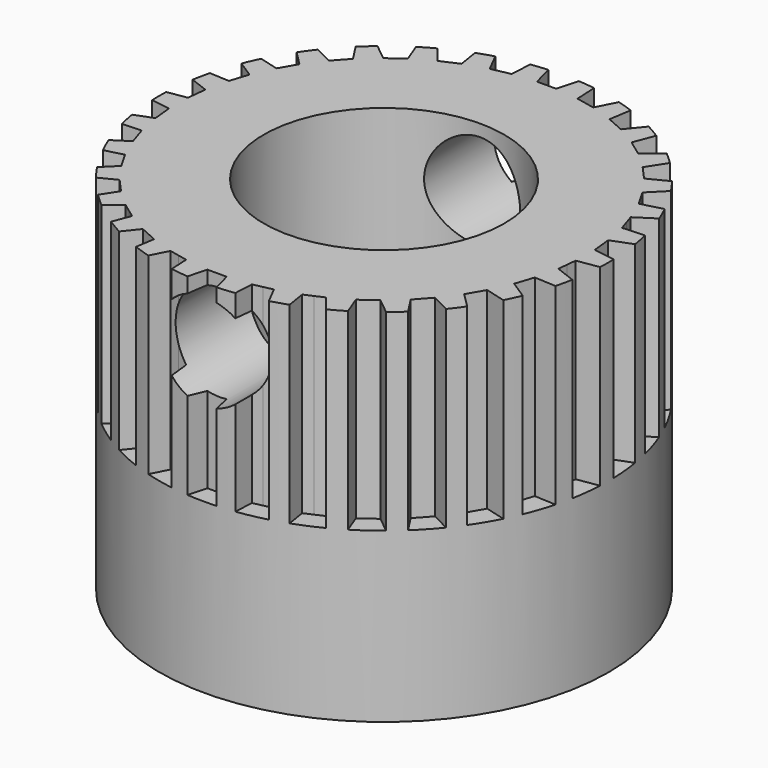
from build123d import *

# Parameters (mm, degrees)
F0_R     = 4.675
F0_R_2   = 2.5
F1_DEPTH = 7.5
F3_DEPTH = 4
F4_R     = 1
F5_DEPTH = 5


# Not quite as in the source:
# - a feature names something its author has since deleted; it is built from what else it names


with BuildPart() as f1:
    # F0 (on Top) → F1 (new body)
    with BuildSketch(Plane.XY):
        Circle(F0_R)
        Circle(F0_R_2, mode=Mode.SUBTRACT)
    extrude(amount=F1_DEPTH)

    # F2 (on face) → F3 (cut)
    with BuildSketch(Plane.XY.offset(7.5)):
        with BuildLine():
            Line((-2.705116146, -3.3310705443), (-3.0094686579, -3.5775303489))
            ThreePointArc((-3.0094686579, -3.5775303489), (-2.7721689372, -3.7643996047), (-2.5232974354, -3.9355552407))
            Line((-2.5232974354, -3.9355552407), (-2.3815093482, -3.5661846452))
            Line((-2.3815093482, -3.5661846452), (-2.5433127471, -3.4486275948))
            Line((-2.5433127471, -3.4486275948), (-2.705116146, -3.3310705443))
        make_face()
        with BuildLine():
            Line((-1.959178461, -3.8160524503), (-2.206532557, -4.12150932))
            ThreePointArc((-2.206532557, -4.12150932), (-1.9353308811, -4.2555985925), (-1.6560241348, -4.3718656275))
            Line((-1.6560241348, -4.3718656275), (-1.593760278, -3.9787471075))
            Line((-1.593760278, -3.9787471075), (-1.7764693695, -3.8973997789))
            Line((-1.7764693695, -3.8973997789), (-1.959178461, -3.8160524503))
        make_face()
        with BuildLine():
            Line((-1.1287078961, -4.1353471727), (-1.3084719445, -4.4881539825))
            ThreePointArc((-1.3084719445, -4.4881539825), (-1.0145824139, -4.5635783685), (-0.7164192765, -4.6197801268))
            Line((-0.7164192765, -4.6197801268), (-0.7374488558, -4.218511849))
            Line((-0.7374488558, -4.218511849), (-0.933078376, -4.1769295108))
            Line((-0.933078376, -4.1769295108), (-1.1287078961, -4.1353471727))
        make_face()
        with BuildLine():
            Line((-0.25, -4.275), (-0.3535915562, -4.6616089509))
            ThreePointArc((-0.3535915562, -4.6616089509), (-0.049245186, -4.6747406251), (0.2553102796, -4.6680233141))
            Line((0.2553102796, -4.6680233141), (0.15, -4.275))
            Line((0.15, -4.275), (-0.05, -4.275))
            Line((-0.05, -4.275), (-0.25, -4.275))
        make_face()
        with BuildLine():
            Line((-3.3339198947, -2.7015974913), (-3.6829835562, -2.8794543103))
            ThreePointArc((-3.6829835562, -2.8794543103), (-3.4894187684, -3.1112026065), (-3.281297254, -3.3299719715))
            Line((-3.281297254, -3.3299719715), (-3.0662676522, -2.9988554215))
            Line((-3.0662676522, -2.9988554215), (-3.2000937734, -2.8502264564))
            Line((-3.2000937734, -2.8502264564), (-3.3339198947, -2.7015974913))
        make_face()
        with BuildLine():
            Line((-3.8181079661, -1.9551442841), (-4.198151087, -2.0569765315))
            ThreePointArc((-4.198151087, -2.0569765315), (-4.0564520262, -2.3239668585), (-3.8977958923, -2.5812423718))
            Line((-3.8977958923, -2.5812423718), (-3.6181079661, -2.3015544457))
            Line((-3.6181079661, -2.3015544457), (-3.7181079661, -2.1283493649))
            Line((-3.7181079661, -2.1283493649), (-3.8181079661, -1.9551442841))
        make_face()
        with BuildLine():
            Line((-4.136519018, -1.1243345099), (-4.5325919451, -1.1450918125))
            ThreePointArc((-4.5325919451, -1.1450918125), (-4.4489051537, -1.4362687538), (-4.3465342095, -1.7214137695))
            Line((-4.3465342095, -1.7214137695), (-4.0129122202, -1.5047571164))
            Line((-4.0129122202, -1.5047571164), (-4.0747156191, -1.3145458132))
            Line((-4.0747156191, -1.3145458132), (-4.136519018, -1.1243345099))
        make_face()
        with BuildLine():
            Line((-4.2752369596, -0.2454785424), (-4.6714275586, -0.1827281161))
            ThreePointArc((-4.6714275586, -0.1827281161), (-4.6496722184, -0.4859766059), (-4.6082522435, -0.7871697783))
            Line((-4.6082522435, -0.7871697783), (-4.2334255742, -0.6432873006))
            Line((-4.2334255742, -0.6432873006), (-4.2543312669, -0.4443829215))
            Line((-4.2543312669, -0.4443829215), (-4.2752369596, -0.2454785424))
        make_face()
        with BuildLine():
            Line((-4.2281991511, 0.6430133953), (-4.6079742635, 0.7887954024))
            ThreePointArc((-4.6079742635, 0.7887954024), (-4.6496441518, 0.4862450633), (-4.6714707885, 0.1816195798))
            Line((-4.6714707885, 0.1816195798), (-4.2700105364, 0.2452046372))
            Line((-4.2700105364, 0.2452046372), (-4.2491048437, 0.4441090163))
            Line((-4.2491048437, 0.4441090163), (-4.2281991511, 0.6430133953))
        make_face()
        with BuildLine():
            Line((-3.9974613705, 1.5023099423), (-4.3441403746, 1.7274459199))
            ThreePointArc((-4.3441403746, 1.7274459199), (-4.4481636875, 1.4385634532), (-4.5329999094, 1.1434757635))
            Line((-4.5329999094, 1.1434757635), (-4.1210681683, 1.1218873357))
            Line((-4.1210681683, 1.1218873357), (-4.0592647694, 1.312098639))
            Line((-4.0592647694, 1.312098639), (-3.9974613705, 1.5023099423))
        make_face()
        with BuildLine():
            Line((-3.5931079661, 2.2948557159), (-3.8904912347, 2.5922389845))
            ThreePointArc((-3.8904912347, 2.5922389845), (-4.0531666787, 2.3296920128), (-4.198151087, 2.0569765315))
            Line((-4.198151087, 2.0569765315), (-3.7931079661, 1.9484455543))
            Line((-3.7931079661, 1.9484455543), (-3.6931079661, 2.1216506351))
            Line((-3.6931079661, 2.1216506351), (-3.5931079661, 2.2948557159))
        make_face()
        with BuildLine():
            Line((-3.0328111218, 2.9860126628), (-3.265954152, 3.3450214464))
            ThreePointArc((-3.265954152, 3.3450214464), (-3.480984636, 3.1206363075), (-3.680631567, 2.8824601069))
            Line((-3.680631567, 2.8824601069), (-3.3004633644, 2.6887547326))
            Line((-3.3004633644, 2.6887547326), (-3.1666372431, 2.8373836977))
            Line((-3.1666372431, 2.8373836977), (-3.0328111218, 2.9860126628))
        make_face()
        with BuildLine():
            Line((-2.3410584985, 3.5455739079), (-2.4971473914, 3.9521993758))
            ThreePointArc((-2.4971473914, 3.9521993758), (-2.7557916794, 3.7764053304), (-3.002104242, 3.5837124774))
            Line((-3.002104242, 3.5837124774), (-2.6646652963, 3.3104598069))
            Line((-2.6646652963, 3.3104598069), (-2.5028618974, 3.4280168574))
            Line((-2.5028618974, 3.4280168574), (-2.3410584985, 3.5455739079))
        make_face()
        with BuildLine():
            Line((-1.5480830051, 3.9490839397), (-1.6173352692, 4.3863255268))
            ThreePointArc((-1.6173352692, 4.3863255268), (-1.9086924345, 4.2676127039), (-2.1914053409, 4.1295723304))
            Line((-2.1914053409, 4.1295723304), (-1.9135011882, 3.7863892824))
            Line((-1.9135011882, 3.7863892824), (-1.7307920966, 3.8677366111))
            Line((-1.7307920966, 3.8677366111), (-1.5480830051, 3.9490839397))
        make_face()
        with BuildLine():
            Line((-0.6885414758, 4.1789074336), (-0.6650340091, 4.6274566197))
            ThreePointArc((-0.6650340091, 4.6274566197), (-0.9764656149, 4.5718858147), (-1.2834259466, 4.4953801663))
            Line((-1.2834259466, 4.4953801663), (-1.0798005161, 4.0957427572))
            Line((-1.0798005161, 4.0957427572), (-0.884170996, 4.1373250954))
            Line((-0.884170996, 4.1373250954), (-0.6885414758, 4.1789074336))
        make_face()
        with BuildLine():
            Line((0, 4.225), (0, 4.675))
            ThreePointArc((0, 4.675), (-0.1589326757, 4.672297658), (-0.3176816122, 4.664193756))
            Line((-0.3176816122, 4.664193756), (-0.2, 4.225))
            Line((-0.2, 4.225), (0, 4.225))
        make_face()
        with BuildLine():
            ThreePointArc((0.3176816122, 4.664193756), (0.1589326757, 4.672297658), (0, 4.675))
            Line((0, 4.675), (0, 4.225))
            Line((0, 4.225), (0.2, 4.225))
            Line((0.2, 4.225), (0.3176816122, 4.664193756))
        make_face()
        with BuildLine():
            ThreePointArc((1.2870955087, 4.4943308903), (0.9775168208, 4.5716611713), (0.6633841691, 4.6276934259))
            Line((0.6633841691, 4.6276934259), (0.6874488558, 4.168511849))
            Line((0.6874488558, 4.168511849), (0.883078376, 4.1269295108))
            Line((0.883078376, 4.1269295108), (1.0787078961, 4.0853471727))
            Line((1.0787078961, 4.0853471727), (1.2870955087, 4.4943308903))
        make_face()
        with BuildLine():
            ThreePointArc((2.1998941634, 4.1250564445), (1.9125739797, 4.2658745612), (1.6162943473, 4.3867091974))
            Line((1.6162943473, 4.3867091974), (1.543760278, 3.9287471075))
            Line((1.543760278, 3.9287471075), (1.7264693695, 3.8473997789))
            Line((1.7264693695, 3.8473997789), (1.909178461, 3.7660524503))
            Line((1.909178461, 3.7660524503), (2.1998941634, 4.1250564445))
        make_face()
        with BuildLine():
            ThreePointArc((3.015224498, 3.572680538), (2.763375727, 3.7708592643), (2.4985414705, 3.9513182003))
            Line((2.4985414705, 3.9513182003), (2.3315093482, 3.5161846452))
            Line((2.3315093482, 3.5161846452), (2.4933127471, 3.3986275948))
            Line((2.4933127471, 3.3986275948), (2.655116146, 3.2810705443))
            Line((2.655116146, 3.2810705443), (3.015224498, 3.572680538))
        make_face()
        with BuildLine():
            ThreePointArc((3.6966467607, 2.8618923332), (3.4918298057, 3.108496358), (3.2705945256, 3.3404844632))
            Line((3.2705945256, 3.3404844632), (3.0162676522, 2.9488554215))
            Line((3.0162676522, 2.9488554215), (3.1500937734, 2.8002264564))
            Line((3.1500937734, 2.8002264564), (3.2839198947, 2.6515974913))
            Line((3.2839198947, 2.6515974913), (3.6966467607, 2.8618923332))
        make_face()
        with BuildLine():
            ThreePointArc((4.2138675521, 2.0245852052), (4.0653705562, 2.308329968), (3.8977958923, 2.5812423718))
            Line((3.8977958923, 2.5812423718), (3.5681079661, 2.2515544457))
            Line((3.5681079661, 2.2515544457), (3.6681079661, 2.0783493649))
            Line((3.6681079661, 2.0783493649), (3.7681079661, 1.9051442841))
            Line((3.7681079661, 1.9051442841), (4.2138675521, 2.0245852052))
        make_face()
        with BuildLine():
            ThreePointArc((4.5441525528, 1.0983180672), (4.4585092177, 1.4061723064), (4.3520358228, 1.7074569386))
            Line((4.3520358228, 1.7074569386), (3.9629122202, 1.4547571164))
            Line((3.9629122202, 1.4547571164), (4.0247156191, 1.2645458132))
            Line((4.0247156191, 1.2645458132), (4.086519018, 1.0743345099))
            Line((4.086519018, 1.0743345099), (4.5441525528, 1.0983180672))
        make_face()
        with BuildLine():
            ThreePointArc((4.673341773, 0.1245057123), (4.6540213184, 0.4423918711), (4.6131030555, 0.7582250323))
            Line((4.6131030555, 0.7582250323), (4.1834255742, 0.5932873006))
            Line((4.1834255742, 0.5932873006), (4.2043312669, 0.3943829215))
            Line((4.2043312669, 0.3943829215), (4.2252369596, 0.1954785424))
            Line((4.2252369596, 0.1954785424), (4.673341773, 0.1245057123))
        make_face()
        with BuildLine():
            ThreePointArc((4.5964194804, -0.8535531385), (4.6437064147, -0.5400145687), (4.6696308942, -0.2239917685))
            Line((4.6696308942, -0.2239917685), (4.2200105364, -0.2952046372))
            Line((4.2200105364, -0.2952046372), (4.1991048437, -0.4941090163))
            Line((4.1991048437, -0.4941090163), (4.1781991511, -0.6930133953))
            Line((4.1781991511, -0.6930133953), (4.5964194804, -0.8535531385))
        make_face()
        with BuildLine():
            ThreePointArc((4.3176228817, -1.7926956383), (4.4286859235, -1.4974531683), (4.5195862819, -1.195393174))
            Line((4.5195862819, -1.195393174), (4.0710681683, -1.1718873357))
            Line((4.0710681683, -1.1718873357), (4.0092647694, -1.362098639))
            Line((4.0092647694, -1.362098639), (3.9474613705, -1.5523099423))
            Line((3.9474613705, -1.5523099423), (4.3176228817, -1.7926956383))
        make_face()
        with BuildLine():
            ThreePointArc((0.6173080827, -4.6340647094), (0.9192758993, -4.5837273938), (1.2173017982, -4.5137347432))
            Line((1.2173017982, -4.5137347432), (1.0298005161, -4.1457427572))
            Line((1.0298005161, -4.1457427572), (0.834170996, -4.1873250954))
            Line((0.834170996, -4.1873250954), (0.6385414758, -4.2289074336))
            Line((0.6385414758, -4.2289074336), (0.6173080827, -4.6340647094))
        make_face()
        with BuildLine():
            ThreePointArc((1.5625539974, -4.4061377651), (1.8491669395, -4.2937404009), (2.1277606959, -4.1627225972))
            Line((2.1277606959, -4.1627225972), (1.8635011882, -3.8363892824))
            Line((1.8635011882, -3.8363892824), (1.6807920966, -3.9177366111))
            Line((1.6807920966, -3.9177366111), (1.4980830051, -3.9990839397))
            Line((1.4980830051, -3.9990839397), (1.5625539974, -4.4061377651))
        make_face()
        with BuildLine():
            ThreePointArc((2.4412913559, -3.9869438817), (2.6999430383, -3.816534107), (2.9467427132, -3.629370797))
            Line((2.9467427132, -3.629370797), (2.6146652963, -3.3604598069))
            Line((2.6146652963, -3.3604598069), (2.4528618974, -3.4780168574))
            Line((2.4528618974, -3.4780168574), (2.2910584985, -3.5955739079))
            Line((2.2910584985, -3.5955739079), (2.4412913559, -3.9869438817))
        make_face()
        with BuildLine():
            ThreePointArc((3.2151897654, -3.3938443943), (3.4341897228, -3.1720602056), (3.6379245568, -2.9361760708))
            Line((3.6379245568, -2.9361760708), (3.2504633644, -2.7387547326))
            Line((3.2504633644, -2.7387547326), (3.1166372431, -2.8873836977))
            Line((3.1166372431, -2.8873836977), (2.9828111218, -3.0360126628))
            Line((2.9828111218, -3.0360126628), (3.2151897654, -3.3938443943))
        make_face()
        with BuildLine():
            ThreePointArc((3.8501044988, -2.6518522486), (4.0192368923, -2.3877520399), (4.1702819153, -2.1129064691))
            Line((4.1702819153, -2.1129064691), (3.7431079661, -1.9984455543))
            Line((3.7431079661, -1.9984455543), (3.6431079661, -2.1716506351))
            Line((3.6431079661, -2.1716506351), (3.5431079661, -2.3448557159))
            Line((3.5431079661, -2.3448557159), (3.8501044988, -2.6518522486))
        make_face()
    extrude(amount=-F3_DEPTH, mode=Mode.SUBTRACT)

    # F4 (on Front) → F5 (cut, symmetric)
    with BuildSketch(Plane.XZ):
        with Locations((0, 6.25)):
            Circle(F4_R)
    extrude(amount=F5_DEPTH, both=True, mode=Mode.SUBTRACT)


solid = f1.part
